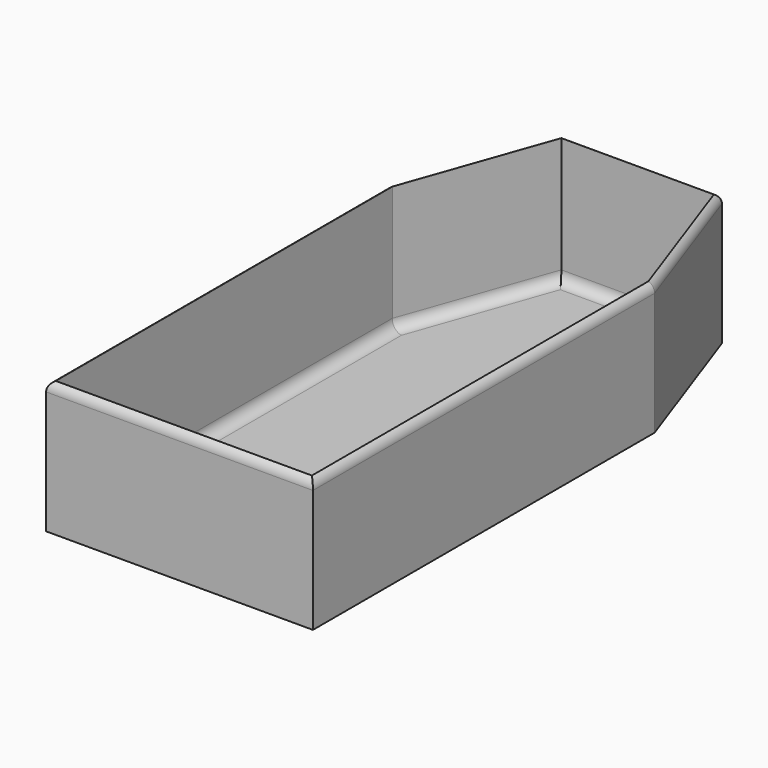
from build123d import *

# Parameters (mm, degrees)
F1_DEPTH    = 63.5
F2_T        = -2.54
F3_R        = 5.08
F4_T1_DEPTH = 110.49
F4_T3_DEPTH = 101.6
F4_T5_DEPTH = 110.49
F4_T7_DEPTH = 237.49
F4_T9_DEPTH = 152.4


# Not quite as in the source:
# - a fillet or chamfer that OpenCascade refuses, or shapes differently, is made with other operations: its cross-section is extruded or revolved along the edge and cut away or added


with BuildPart() as f1:
    # F0 (on Top) → F1 (new body)
    with BuildSketch(Plane.XY):
        Polygon((-32.2156401169, 127.5564689514), (-57.6156401169, 55.7144199828), (-57.6156401169, -147.4855800172), (69.3843598831, -147.4855800172), (69.3843598831, 55.7144199828), (43.9843598831, 127.5564689514), align=None)
    extrude(amount=F1_DEPTH)

    # F2
    f2_openings = [f1.faces().sort_by_distance(p)[0] for p in [
        (5.88436, -16.224771, 63.5),
    ]]
    offset(amount=F2_T, openings=f2_openings)

    # F3
    f3_edges = [f1.edges().sort_by_distance(p)[0] for p in [
        (54.516334, 90.147547, 2.54),
        (5.88436, 125.016469, 2.54),
        (-42.747615, 90.147547, 2.54),
        (-55.07564, -44.833478, 2.54),
        (5.88436, -144.94558, 2.54),
        (66.84436, -44.833478, 2.54),
    ]]
    fillet(f3_edges, radius=F3_R)

    # F4: fillet of radius 5.08 on 6 edges, made by hand

    # F4_s2 → F4_t1 (cut)
    with BuildSketch(Plane(origin=(40.7409485113, 115.2328038573, 0), x_dir=(0, 0, 1), z_dir=(-0.3333333333, -0.9428090416, 0))):
        with BuildLine():
            ThreePointArc((63.5, 67.8120197664), (62.0121024484, 71.4041222148), (58.42, 72.8920197664))
            Line((58.42, 72.8920197664), (63.5, 72.8920197664))
            Line((63.5, 72.8920197664), (63.5, 67.8120197664))
        make_face()
    extrude(amount=F4_T1_DEPTH, mode=Mode.SUBTRACT)

    # F4_s4 → F4_t3 (cut)
    with BuildSketch(Plane.YZ.offset(-44.9156401169)):
        with BuildLine():
            ThreePointArc((122.4764689514, 63.5), (126.0685713998, 62.0121024484), (127.5564689514, 58.42))
            Line((127.5564689514, 58.42), (127.5564689514, 63.5))
            Line((127.5564689514, 63.5), (122.4764689514, 63.5))
        make_face()
    extrude(amount=F4_T3_DEPTH, mode=Mode.SUBTRACT)

    # F4_s6 → F4_t5 (cut)
    with BuildSketch(Plane(origin=(-2.6033129818, 7.3632810518, 0), x_dir=(0, 0, 1), z_dir=(-0.3333333333, 0.9428090416, 0))):
        with BuildLine():
            ThreePointArc((63.5, 78.9076751698), (62.0121024484, 82.4997776182), (58.42, 83.9876751698))
            Line((58.42, 83.9876751698), (63.5, 83.9876751698))
            Line((63.5, 83.9876751698), (63.5, 78.9076751698))
        make_face()
    extrude(amount=F4_T5_DEPTH, mode=Mode.SUBTRACT)

    # F4_s8 → F4_t7 (cut)
    with BuildSketch(Plane.XZ.offset(-77.3044199828)):
        with BuildLine():
            ThreePointArc((-52.5356401169, 63.5), (-56.1277425653, 62.0121024484), (-57.6156401169, 58.42))
            Line((-57.6156401169, 58.42), (-57.6156401169, 63.5))
            Line((-57.6156401169, 63.5), (-52.5356401169, 63.5))
        make_face()
        with BuildLine():
            ThreePointArc((64.3043598831, 63.5), (67.8964623315, 62.0121024484), (69.3843598831, 58.42))
            Line((69.3843598831, 58.42), (69.3843598831, 63.5))
            Line((69.3843598831, 63.5), (64.3043598831, 63.5))
        make_face()
    extrude(amount=F4_T7_DEPTH, mode=Mode.SUBTRACT)

    # F4_s10 → F4_t9 (cut)
    with BuildSketch(Plane.YZ.offset(-70.3156401169)):
        with BuildLine():
            ThreePointArc((-142.4055800172, 63.5), (-145.9976824656, 62.0121024484), (-147.4855800172, 58.42))
            Line((-147.4855800172, 58.42), (-147.4855800172, 63.5))
            Line((-147.4855800172, 63.5), (-142.4055800172, 63.5))
        make_face()
    extrude(amount=F4_T9_DEPTH, mode=Mode.SUBTRACT)


solid = f1.part
